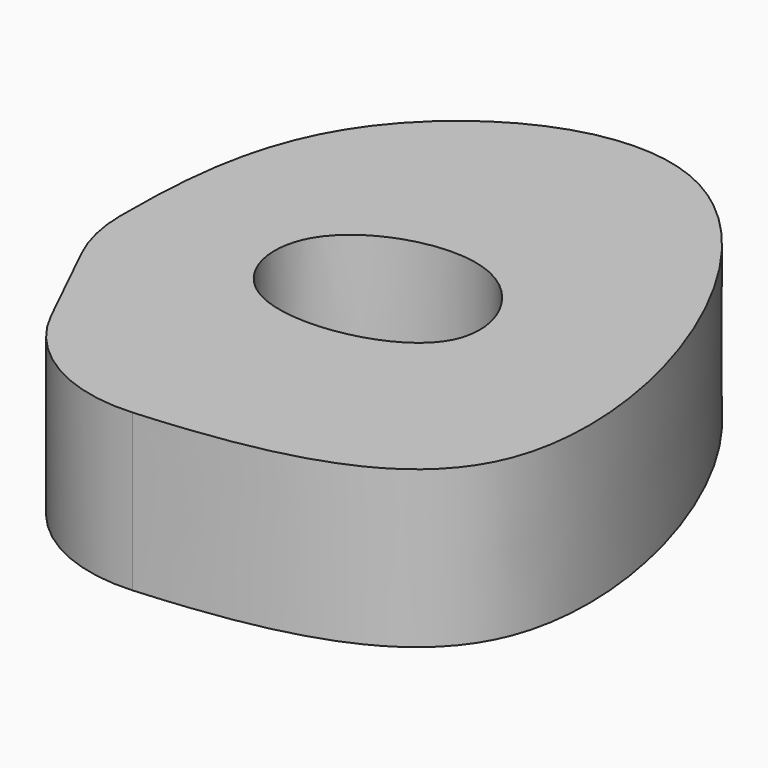
from build123d import *

# Parameters (mm, degrees)
F1_DEPTH = 25.4
F3_DEPTH = 104.902


with BuildPart() as f1:
    # F0 (on Top) → F1 (new body)
    with BuildSketch(Plane.XY):
        with BuildLine():
            add(Edge.make_bspline(
                [(-46.0991912945, -10.5556205251), (-46.0990739821, 3.1401170204), (-44.2047112287, 31.9258238437), (14.0830478954, 63.0674394607), (53.6330898009, -41.1624333533), (9.8180946284, -50.2912053998), (-11.1846181743, -51.7680321244)],
                knots=[0.027765762, 0.027765762, 0.027765762, 0.027765762, 0.2204439576, 0.441423506, 0.7331940213, 0.9435786765, 0.9435786765, 0.9435786765, 0.9435786765], degree=3))
            ThreePointArc((-46.0991912945, -10.5556205251), (-45.4496236559, -16.2633855485), (-43.5340489335, -21.6792043382))
            add(Edge.make_bspline(
                [(-35.8011031231, -37.5539595869), (-38.3787517266, -32.262374504), (-40.95640033, -26.9707894211), (-43.5340489335, -21.6792043382)],
                knots=[16.7567995992, 16.7567995992, 16.7567995992, 16.7567995992, 34.4148375738, 34.4148375738, 34.4148375738, 34.4148375738], degree=3))
            ThreePointArc((-35.8011031231, -37.5539595869), (-25.6674104446, -48.4269659659), (-11.1846181743, -51.7680321244))
        make_face()
    extrude(amount=F1_DEPTH)

    # F2 (on face) → F3 (cut)
    with BuildSketch(Plane.XY.offset(25.4)):
        with BuildLine():
            add(Edge.make_bspline(
                [(-23.2676491141, 0), (-19.3057295103, 6.5657089804), (2.4302119089, 13.2204227766), (16.0169378818, -15.8120767234), (-22.0808563681, -22.9530178694), (-26.6284403137, -5.5695165896), (-23.2676491141, 0)],
                knots=[0, 0, 0, 0, 0.2635074208, 0.4999073959, 0.7764736519, 1, 1, 1, 1], degree=3))
        make_face()
    extrude(amount=-F3_DEPTH, mode=Mode.SUBTRACT)


solid = f1.part
